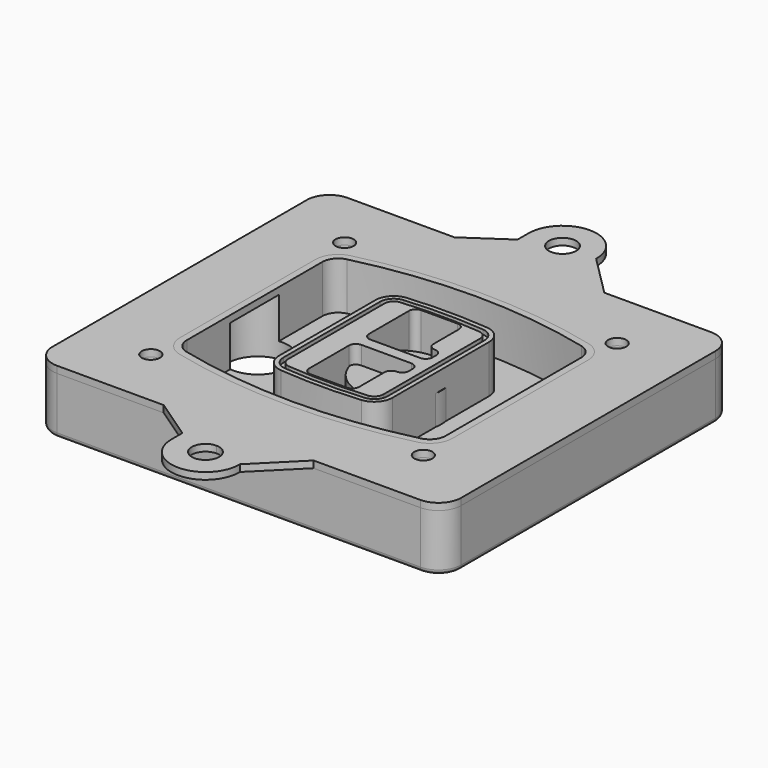
from build123d import *

# Parameters (mm, degrees)
F0_R      = 4
F1_DEPTH  = 25
F2_DEPTH  = 3
F3_DEPTH  = 18
F5_DEPTH  = 21
F6_DEPTH  = 2
F8_DEPTH  = 20
F9_DEPTH  = 16
F10_DEPTH = 25
F7_R      = 6
F7_R_2    = 4
F11_DEPTH = 6
F13_DEPTH = 9
F15_R     = 2
F16_R     = 4
F17_DEPTH = 3


# Not quite as in the source:
# - a feature of the source that left no trace in its solid (it failed there, or was rolled back) is left out
# - a feature names something its author has since deleted; it is built from what else it names


with BuildPart() as f1:
    # F0 (on Top) → F1 (new body)
    with BuildSketch(Plane.XY):
        with BuildLine():
            ThreePointArc((-90, -70), (-87.0710678119, -77.0710678119), (-80, -80))
            Line((-80, -80), (80, -80))
            ThreePointArc((80, -80), (87.0710678119, -77.0710678119), (90, -70))
            Line((90, -70), (90, 70))
            ThreePointArc((90, 70), (87.0710678119, 77.0710678119), (80, 80))
            Line((80, 80), (-80, 80))
            ThreePointArc((-80, 80), (-87.0710678119, 77.0710678119), (-90, 70))
            Line((-90, 70), (-90, -70))
        make_face()
        with Locations((-60, -53.3333333333)):
            Circle(F0_R, mode=Mode.SUBTRACT)
        with Locations((60, -53.3333333333)):
            Circle(F0_R, mode=Mode.SUBTRACT)
        with BuildLine():
            ThreePointArc((-64, 37.2990447398), (-61.0143011354, 45.9411029726), (-53.3306899286, 50.8970778549))
            ThreePointArc((-53.3306899286, 50.8970778549), (0, 57.3333333333), (53.3306899286, 50.8970778549))
            ThreePointArc((53.3306899286, 50.8970778549), (61.0143011354, 45.9411029726), (64, 37.2990447398))
            Line((64, 37.2990447398), (64, -37.2990447398))
            ThreePointArc((64, -37.2990447398), (61.0143011354, -45.9411029726), (53.3306899286, -50.8970778549))
            ThreePointArc((53.3306899286, -50.8970778549), (0, -57.3333333333), (-53.3306899286, -50.8970778549))
            ThreePointArc((-53.3306899286, -50.8970778549), (-61.0143011354, -45.9411029726), (-64, -37.2990447398))
            Line((-64, -37.2990447398), (-64, 37.2990447398))
        make_face(mode=Mode.SUBTRACT)
        with Locations((-60, 53.3333333333)):
            Circle(F0_R, mode=Mode.SUBTRACT)
        with Locations((60, 53.3333333333)):
            Circle(F0_R, mode=Mode.SUBTRACT)
        with BuildLine():
            ThreePointArc((53.3306899286, 50.8970778549), (0, 57.3333333333), (-53.3306899286, 50.8970778549))
            ThreePointArc((-53.3306899286, 50.8970778549), (-61.0143011354, 45.9411029726), (-64, 37.2990447398))
            Line((-64, 37.2990447398), (-64, -37.2990447398))
            ThreePointArc((-64, -37.2990447398), (-61.0143011354, -45.9411029726), (-53.3306899286, -50.8970778549))
            ThreePointArc((-53.3306899286, -50.8970778549), (0, -57.3333333333), (53.3306899286, -50.8970778549))
            ThreePointArc((53.3306899286, -50.8970778549), (61.0143011354, -45.9411029726), (64, -37.2990447398))
            Line((64, -37.2990447398), (64, 37.2990447398))
            ThreePointArc((64, 37.2990447398), (61.0143011354, 45.9411029726), (53.3306899286, 50.8970778549))
        make_face()
        with BuildLine():
            Line((-60, -37.2990447398), (-60, 37.2990447398))
            ThreePointArc((-60, 37.2990447398), (-57.8673579538, 43.4719434775), (-52.3790642347, 47.0119255363))
            ThreePointArc((-52.3790642347, 47.0119255363), (0, 53.3333333333), (52.3790642347, 47.0119255363))
            ThreePointArc((52.3790642347, 47.0119255363), (57.8673579538, 43.4719434775), (60, 37.2990447398))
            Line((60, 37.2990447398), (60, -37.2990447398))
            ThreePointArc((60, -37.2990447398), (57.8673579538, -43.4719434775), (52.3790642347, -47.0119255363))
            ThreePointArc((52.3790642347, -47.0119255363), (0, -53.3333333333), (-52.3790642347, -47.0119255363))
            ThreePointArc((-52.3790642347, -47.0119255363), (-57.8673579538, -43.4719434775), (-60, -37.2990447398))
        make_face(mode=Mode.SUBTRACT)
        with BuildLine():
            ThreePointArc((-52.3790642347, 47.0119255363), (-57.8673579538, 43.4719434775), (-60, 37.2990447398))
            Line((-60, 37.2990447398), (-60, -37.2990447398))
            ThreePointArc((-60, -37.2990447398), (-57.8673579538, -43.4719434775), (-52.3790642347, -47.0119255363))
            ThreePointArc((-52.3790642347, -47.0119255363), (0, -53.3333333333), (52.3790642347, -47.0119255363))
            ThreePointArc((52.3790642347, -47.0119255363), (57.8673579538, -43.4719434775), (60, -37.2990447398))
            Line((60, -37.2990447398), (60, 37.2990447398))
            ThreePointArc((60, 37.2990447398), (57.8673579538, 43.4719434775), (52.3790642347, 47.0119255363))
            ThreePointArc((52.3790642347, 47.0119255363), (0, 53.3333333333), (-52.3790642347, 47.0119255363))
        make_face()
        with BuildLine():
            ThreePointArc((51.6653449643, 44.0980612973), (55.5071505677, 41.6200738562), (57, 37.2990447398))
            Line((57, 37.2990447398), (57, -37.2990447398))
            ThreePointArc((57, -37.2990447398), (55.5071505677, -41.6200738562), (51.6653449643, -44.0980612973))
            ThreePointArc((51.6653449643, -44.0980612973), (0, -50.3333333333), (-51.6653449643, -44.0980612973))
            ThreePointArc((-51.6653449643, -44.0980612973), (-55.5071505677, -41.6200738562), (-57, -37.2990447398))
            Line((-57, -37.2990447398), (-57, 37.2990447398))
            ThreePointArc((-57, 37.2990447398), (-55.5071505677, 41.6200738562), (-51.6653449643, 44.0980612973))
            ThreePointArc((-51.6653449643, 44.0980612973), (0, 50.3333333333), (51.6653449643, 44.0980612973))
        make_face(mode=Mode.SUBTRACT)
        with BuildLine():
            Line((57, -37.2990447398), (57, 37.2990447398))
            ThreePointArc((57, 37.2990447398), (55.5071505677, 41.6200738562), (51.6653449643, 44.0980612973))
            ThreePointArc((51.6653449643, 44.0980612973), (0, 50.3333333333), (-51.6653449643, 44.0980612973))
            ThreePointArc((-51.6653449643, 44.0980612973), (-55.5071505677, 41.6200738562), (-57, 37.2990447398))
            Line((-57, 37.2990447398), (-57, -37.2990447398))
            ThreePointArc((-57, -37.2990447398), (-55.5071505677, -41.6200738562), (-51.6653449643, -44.0980612973))
            ThreePointArc((-51.6653449643, -44.0980612973), (0, -50.3333333333), (51.6653449643, -44.0980612973))
            ThreePointArc((51.6653449643, -44.0980612973), (55.5071505677, -41.6200738562), (57, -37.2990447398))
        make_face()
    extrude(amount=-F1_DEPTH)

    # F0 (on Top) → F2 (join)
    with BuildSketch(Plane.XY):
        with BuildLine():
            ThreePointArc((-52.3790642347, 47.0119255363), (-57.8673579538, 43.4719434775), (-60, 37.2990447398))
            Line((-60, 37.2990447398), (-60, -37.2990447398))
            ThreePointArc((-60, -37.2990447398), (-57.8673579538, -43.4719434775), (-52.3790642347, -47.0119255363))
            ThreePointArc((-52.3790642347, -47.0119255363), (0, -53.3333333333), (52.3790642347, -47.0119255363))
            ThreePointArc((52.3790642347, -47.0119255363), (57.8673579538, -43.4719434775), (60, -37.2990447398))
            Line((60, -37.2990447398), (60, 37.2990447398))
            ThreePointArc((60, 37.2990447398), (57.8673579538, 43.4719434775), (52.3790642347, 47.0119255363))
            ThreePointArc((52.3790642347, 47.0119255363), (0, 53.3333333333), (-52.3790642347, 47.0119255363))
        make_face()
        with BuildLine():
            ThreePointArc((51.6653449643, 44.0980612973), (55.5071505677, 41.6200738562), (57, 37.2990447398))
            Line((57, 37.2990447398), (57, -37.2990447398))
            ThreePointArc((57, -37.2990447398), (55.5071505677, -41.6200738562), (51.6653449643, -44.0980612973))
            ThreePointArc((51.6653449643, -44.0980612973), (0, -50.3333333333), (-51.6653449643, -44.0980612973))
            ThreePointArc((-51.6653449643, -44.0980612973), (-55.5071505677, -41.6200738562), (-57, -37.2990447398))
            Line((-57, -37.2990447398), (-57, 37.2990447398))
            ThreePointArc((-57, 37.2990447398), (-55.5071505677, 41.6200738562), (-51.6653449643, 44.0980612973))
            ThreePointArc((-51.6653449643, 44.0980612973), (0, 50.3333333333), (51.6653449643, 44.0980612973))
        make_face(mode=Mode.SUBTRACT)
    extrude(amount=F2_DEPTH)

    # F0 (on Top) → F3 (cut)
    with BuildSketch(Plane.XY):
        with BuildLine():
            Line((57, -37.2990447398), (57, 37.2990447398))
            ThreePointArc((57, 37.2990447398), (55.5071505677, 41.6200738562), (51.6653449643, 44.0980612973))
            ThreePointArc((51.6653449643, 44.0980612973), (0, 50.3333333333), (-51.6653449643, 44.0980612973))
            ThreePointArc((-51.6653449643, 44.0980612973), (-55.5071505677, 41.6200738562), (-57, 37.2990447398))
            Line((-57, 37.2990447398), (-57, -37.2990447398))
            ThreePointArc((-57, -37.2990447398), (-55.5071505677, -41.6200738562), (-51.6653449643, -44.0980612973))
            ThreePointArc((-51.6653449643, -44.0980612973), (0, -50.3333333333), (51.6653449643, -44.0980612973))
            ThreePointArc((51.6653449643, -44.0980612973), (55.5071505677, -41.6200738562), (57, -37.2990447398))
        make_face()
    extrude(amount=-F3_DEPTH, mode=Mode.SUBTRACT)

    # F4 (on face) → F5 (join, through all)
    with BuildSketch(Plane.XY.offset(3)):
        with BuildLine():
            ThreePointArc((-25, -26.587695628), (-22.8992979869, -31.9912392117), (-17.7004291845, -34.5569740744))
            ThreePointArc((-17.7004291845, -34.5569740744), (0, -35.3333333333), (17.7004291845, -34.5569740744))
            ThreePointArc((17.7004291845, -34.5569740744), (22.8992979869, -31.9912392117), (25, -26.587695628))
            Line((25, -26.587695628), (25, 26.587695628))
            ThreePointArc((25, 26.587695628), (22.8992979869, 31.9912392117), (17.7004291845, 34.5569740744))
            ThreePointArc((17.7004291845, 34.5569740744), (0, 35.3333333333), (-17.7004291845, 34.5569740744))
            ThreePointArc((-17.7004291845, 34.5569740744), (-22.8992979869, 31.9912392117), (-25, 26.587695628))
            Line((-25, 26.587695628), (-25, -26.587695628))
        make_face()
        with BuildLine():
            ThreePointArc((17.5253218884, 32.5646544628), (21.4244734902, 30.6403533158), (23, 26.587695628))
            Line((23, 26.587695628), (23, -26.587695628))
            ThreePointArc((23, -26.587695628), (21.4244734902, -30.6403533158), (17.5253218884, -32.5646544628))
            ThreePointArc((17.5253218884, -32.5646544628), (0, -33.3333333333), (-17.5253218884, -32.5646544628))
            ThreePointArc((-17.5253218884, -32.5646544628), (-21.4244734902, -30.6403533158), (-23, -26.587695628))
            Line((-23, -26.587695628), (-23, 26.587695628))
            ThreePointArc((-23, 26.587695628), (-21.4244734902, 30.6403533158), (-17.5253218884, 32.5646544628))
            ThreePointArc((-17.5253218884, 32.5646544628), (0, 33.3333333333), (17.5253218884, 32.5646544628))
        make_face(mode=Mode.SUBTRACT)
        with BuildLine():
            Line((23, -26.587695628), (23, 26.587695628))
            ThreePointArc((23, 26.587695628), (21.4244734902, 30.6403533158), (17.5253218884, 32.5646544628))
            ThreePointArc((17.5253218884, 32.5646544628), (0, 33.3333333333), (-17.5253218884, 32.5646544628))
            ThreePointArc((-17.5253218884, 32.5646544628), (-21.4244734902, 30.6403533158), (-23, 26.587695628))
            Line((-23, 26.587695628), (-23, -26.587695628))
            ThreePointArc((-23, -26.587695628), (-21.4244734902, -30.6403533158), (-17.5253218884, -32.5646544628))
            ThreePointArc((-17.5253218884, -32.5646544628), (0, -33.3333333333), (17.5253218884, -32.5646544628))
            ThreePointArc((17.5253218884, -32.5646544628), (21.4244734902, -30.6403533158), (23, -26.587695628))
        make_face()
        with BuildLine():
            ThreePointArc((17.3502145923, 30.5723348512), (19.9496489934, 29.2894674198), (21, 26.587695628))
            Line((21, 26.587695628), (21, -26.587695628))
            ThreePointArc((21, -26.587695628), (19.9496489934, -29.2894674198), (17.3502145923, -30.5723348512))
            ThreePointArc((17.3502145923, -30.5723348512), (0, -31.3333333333), (-17.3502145923, -30.5723348512))
            ThreePointArc((-17.3502145923, -30.5723348512), (-19.9496489934, -29.2894674198), (-21, -26.587695628))
            Line((-21, -26.587695628), (-21, 26.587695628))
            ThreePointArc((-21, 26.587695628), (-19.9496489934, 29.2894674198), (-17.3502145923, 30.5723348512))
            ThreePointArc((-17.3502145923, 30.5723348512), (0, 31.3333333333), (17.3502145923, 30.5723348512))
        make_face(mode=Mode.SUBTRACT)
        with BuildLine():
            Line((21, -26.587695628), (21, 26.587695628))
            ThreePointArc((21, 26.587695628), (19.9496489934, 29.2894674198), (17.3502145923, 30.5723348512))
            ThreePointArc((17.3502145923, 30.5723348512), (0, 31.3333333333), (-17.3502145923, 30.5723348512))
            ThreePointArc((-17.3502145923, 30.5723348512), (-19.9496489934, 29.2894674198), (-21, 26.587695628))
            Line((-21, 26.587695628), (-21, -26.587695628))
            ThreePointArc((-21, -26.587695628), (-19.9496489934, -29.2894674198), (-17.3502145923, -30.5723348512))
            ThreePointArc((-17.3502145923, -30.5723348512), (0, -31.3333333333), (17.3502145923, -30.5723348512))
            ThreePointArc((17.3502145923, -30.5723348512), (19.9496489934, -29.2894674198), (21, -26.587695628))
        make_face()
        with BuildLine():
            Line((-8, -2.5), (14, -2.5))
            ThreePointArc((14, -2.5), (16.1213203436, -3.3786796564), (17, -5.5))
            Line((17, -5.5), (17, -7.5))
            ThreePointArc((17, -7.5), (16.1213203436, -9.6213203436), (14, -10.5))
            ThreePointArc((14, -10.5), (11.8786796564, -11.3786796564), (11, -13.5))
            Line((11, -13.5), (11, -27.5))
            ThreePointArc((11, -27.5), (10.1213203436, -29.6213203436), (8, -30.5))
            Line((8, -30.5), (-8, -30.5))
            ThreePointArc((-8, -30.5), (-10.1213203436, -29.6213203436), (-11, -27.5))
            Line((-11, -27.5), (-11, -5.5))
            ThreePointArc((-11, -5.5), (-10.1213203436, -3.3786796564), (-8, -2.5))
        make_face(mode=Mode.SUBTRACT)
        with BuildLine():
            ThreePointArc((-8, 2.5), (-10.1213203436, 3.3786796564), (-11, 5.5))
            Line((-11, 5.5), (-11, 27.5))
            ThreePointArc((-11, 27.5), (-10.1213203436, 29.6213203436), (-8, 30.5))
            Line((-8, 30.5), (8, 30.5))
            ThreePointArc((8, 30.5), (10.1213203436, 29.6213203436), (11, 27.5))
            Line((11, 27.5), (11, 13.5))
            ThreePointArc((11, 13.5), (11.8786796564, 11.3786796564), (14, 10.5))
            ThreePointArc((14, 10.5), (16.1213203436, 9.6213203436), (17, 7.5))
            Line((17, 7.5), (17, 5.5))
            ThreePointArc((17, 5.5), (16.1213203436, 3.3786796564), (14, 2.5))
            Line((14, 2.5), (-8, 2.5))
        make_face(mode=Mode.SUBTRACT)
    extrude(amount=-F5_DEPTH)

    # F4 (on face) → F6 (cut)
    with BuildSketch(Plane.XY.offset(3)):
        with BuildLine():
            Line((23, -26.587695628), (23, 26.587695628))
            ThreePointArc((23, 26.587695628), (21.4244734902, 30.6403533158), (17.5253218884, 32.5646544628))
            ThreePointArc((17.5253218884, 32.5646544628), (0, 33.3333333333), (-17.5253218884, 32.5646544628))
            ThreePointArc((-17.5253218884, 32.5646544628), (-21.4244734902, 30.6403533158), (-23, 26.587695628))
            Line((-23, 26.587695628), (-23, -26.587695628))
            ThreePointArc((-23, -26.587695628), (-21.4244734902, -30.6403533158), (-17.5253218884, -32.5646544628))
            ThreePointArc((-17.5253218884, -32.5646544628), (0, -33.3333333333), (17.5253218884, -32.5646544628))
            ThreePointArc((17.5253218884, -32.5646544628), (21.4244734902, -30.6403533158), (23, -26.587695628))
        make_face()
        with BuildLine():
            ThreePointArc((17.3502145923, 30.5723348512), (19.9496489934, 29.2894674198), (21, 26.587695628))
            Line((21, 26.587695628), (21, -26.587695628))
            ThreePointArc((21, -26.587695628), (19.9496489934, -29.2894674198), (17.3502145923, -30.5723348512))
            ThreePointArc((17.3502145923, -30.5723348512), (0, -31.3333333333), (-17.3502145923, -30.5723348512))
            ThreePointArc((-17.3502145923, -30.5723348512), (-19.9496489934, -29.2894674198), (-21, -26.587695628))
            Line((-21, -26.587695628), (-21, 26.587695628))
            ThreePointArc((-21, 26.587695628), (-19.9496489934, 29.2894674198), (-17.3502145923, 30.5723348512))
            ThreePointArc((-17.3502145923, 30.5723348512), (0, 31.3333333333), (17.3502145923, 30.5723348512))
        make_face(mode=Mode.SUBTRACT)
    extrude(amount=-F6_DEPTH, mode=Mode.SUBTRACT)

    # F7 (on face) → F8 (join)
    with BuildSketch(Plane(origin=(0, 0, -25), x_dir=(1, 0, 0), z_dir=(0, 0, -1))):
        with BuildLine():
            ThreePointArc((-6.71157564, 0), (6.7567035675, 13.4682792075), (20.224982775, 0))
            Line((20.224982775, 0), (25.224982775, 0))
            ThreePointArc((25.224982775, 0), (6.7567035675, 18.4682792075), (-11.71157564, 0))
            Line((-11.71157564, 0), (-6.71157564, 0))
        make_face()
        with BuildLine():
            Line((-6.71157564, 0), (20.224982775, 0))
            ThreePointArc((20.224982775, 0), (6.7567035675, 13.4682792075), (-6.71157564, 0))
        make_face()
        with BuildLine():
            ThreePointArc((-6.71157564, 0), (6.7567035675, -13.4682792075), (20.224982775, 0))
            Line((20.224982775, 0), (-6.71157564, 0))
        make_face()
        with BuildLine():
            Line((25.224982775, 0), (20.224982775, 0))
            ThreePointArc((20.224982775, 0), (6.7567035675, -13.4682792075), (-6.71157564, 0))
            Line((-6.71157564, 0), (-11.71157564, 0))
            ThreePointArc((-11.71157564, 0), (6.7567035675, -18.4682792075), (25.224982775, 0))
        make_face()
    extrude(amount=-F8_DEPTH)

    # F7 (on face) → F9 (cut)
    with BuildSketch(Plane(origin=(0, 0, -25), x_dir=(1, 0, 0), z_dir=(0, 0, -1))):
        with BuildLine():
            Line((-6.71157564, 0), (20.224982775, 0))
            ThreePointArc((20.224982775, 0), (6.7567035675, 13.4682792075), (-6.71157564, 0))
        make_face()
        with BuildLine():
            ThreePointArc((-6.71157564, 0), (6.7567035675, -13.4682792075), (20.224982775, 0))
            Line((20.224982775, 0), (-6.71157564, 0))
        make_face()
    extrude(amount=-F9_DEPTH, mode=Mode.SUBTRACT)

    # F7 (on face) → F10 (cut)
    with BuildSketch(Plane(origin=(0, 0, -25), x_dir=(1, 0, 0), z_dir=(0, 0, -1))):
        with BuildLine():
            Line((-69.0318229325, 0), (-42.0952645175, 0))
            ThreePointArc((-42.0952645175, 0), (-55.563543725, 13.4682792075), (-69.0318229325, 0))
        make_face()
        with BuildLine():
            ThreePointArc((-69.0318229325, 0), (-55.563543725, -13.4682792075), (-42.0952645175, 0))
            Line((-42.0952645175, 0), (-69.0318229325, 0))
        make_face()
    extrude(amount=-F10_DEPTH, mode=Mode.SUBTRACT)

    # F7 (on face) → F11 (cut)
    with BuildSketch(Plane(origin=(0, 0, -25), x_dir=(1, 0, 0), z_dir=(0, 0, -1))):
        with Locations((60, -53.3333333333)):
            Circle(F7_R)
        with Locations((60, -53.3333333333)):
            Circle(F7_R_2, mode=Mode.SUBTRACT)
        with Locations((-60, -53.3333333333)):
            Circle(F7_R)
        with Locations((-60, -53.3333333333)):
            Circle(F7_R_2, mode=Mode.SUBTRACT)
        with Locations((-60, 53.3333333333)):
            Circle(F7_R)
        with Locations((-60, 53.3333333333)):
            Circle(F7_R_2, mode=Mode.SUBTRACT)
        with Locations((60, 53.3333333333)):
            Circle(F7_R)
        with Locations((60, 53.3333333333)):
            Circle(F7_R_2, mode=Mode.SUBTRACT)
    extrude(amount=-F11_DEPTH, mode=Mode.SUBTRACT)

    # F12 (on face) → F13 (cut, through all)
    with BuildSketch(Plane(origin=(0, 0, -9), x_dir=(1, 0, 0), z_dir=(0, 0, -1))):
        with BuildLine():
            ThreePointArc((20.224982775, 0), (20.1663399806, 1.2554664788), (19.9909222755, 2.5))
            Line((19.9909222755, 2.5), (14, 2.5))
            ThreePointArc((14, 2.5), (16.1213203436, 3.3786796564), (17, 5.5))
            Line((17, 5.5), (17, 7.5))
            ThreePointArc((17, 7.5), (16.1213203436, 9.6213203436), (14, 10.5))
            ThreePointArc((14, 10.5), (12.1627255951, 11.1284134507), (11.0951631559, 12.750384826))
            ThreePointArc((11.0951631559, 12.750384826), (11.0476113807, 12.7664660322), (11, 12.7823698976))
            Line((11, 12.7823698976), (11, -12.7823698976))
            ThreePointArc((11, -12.7823698976), (11.0476113807, -12.7664660322), (11.0951631559, -12.750384826))
            ThreePointArc((11.0951631559, -12.750384826), (12.1627255951, -11.1284134507), (14, -10.5))
            ThreePointArc((14, -10.5), (16.1213203436, -9.6213203436), (17, -7.5))
            Line((17, -7.5), (17, -5.5))
            ThreePointArc((17, -5.5), (16.1213203436, -3.3786796564), (14, -2.5))
            Line((14, -2.5), (19.9909222755, -2.5))
            ThreePointArc((19.9909222755, -2.5), (20.1663399806, -1.2554664788), (20.224982775, 0))
        make_face()
    extrude(amount=F13_DEPTH, mode=Mode.SUBTRACT)

    # F15
    f15_edges = [f1.edges().sort_by_distance(p)[0] for p in [
        (0, -80, -25),
        (-87.071068, -77.071068, -25),
        (-90, 0, -25),
        (-87.071068, 77.071068, -25),
        (87.071068, -77.071068, -25),
        (0, 80, -25),
        (90, 0, -25),
        (87.071068, 77.071068, -25),
    ]]
    fillet(f15_edges, radius=F15_R)


with BuildPart() as f17:
    # F16 (on face) → F17 (new body, through all)
    with BuildSketch(Plane.XY):
        with BuildLine():
            Line((-33, 80), (-80, 80))
            ThreePointArc((-80, 80), (-87.0710678119, 77.0710678119), (-90, 70))
            Line((-90, 70), (-90, -70))
            ThreePointArc((-90, -70), (-87.0710678119, -77.0710678119), (-80, -80))
            Line((-80, -80), (-33, -80))
            Line((-33, -80), (0, -80))
            Line((0, -80), (33, -80))
            Line((33, -80), (80, -80))
            ThreePointArc((80, -80), (87.0710678119, -77.0710678119), (90, -70))
            Line((90, -70), (90, 70))
            ThreePointArc((90, 70), (87.0710678119, 77.0710678119), (80, 80))
            Line((80, 80), (33, 80))
            Line((33, 80), (0, 80))
            Line((0, 80), (-33, 80))
        make_face()
        with Locations((-60, -53.3333333333)):
            Circle(F16_R, mode=Mode.SUBTRACT)
        with BuildLine():
            ThreePointArc((52.3790642347, -47.0119255363), (0, -53.3333333333), (-52.3790642347, -47.0119255363))
            ThreePointArc((-52.3790642347, -47.0119255363), (-57.8673579538, -43.4719434775), (-60, -37.2990447398))
            Line((-60, -37.2990447398), (-60, 37.2990447398))
            ThreePointArc((-60, 37.2990447398), (-57.8673579538, 43.4719434775), (-52.3790642347, 47.0119255363))
            ThreePointArc((-52.3790642347, 47.0119255363), (0, 53.3333333333), (52.3790642347, 47.0119255363))
            ThreePointArc((52.3790642347, 47.0119255363), (57.8673579538, 43.4719434775), (60, 37.2990447398))
            Line((60, 37.2990447398), (60, -37.2990447398))
            ThreePointArc((60, -37.2990447398), (57.8673579538, -43.4719434775), (52.3790642347, -47.0119255363))
        make_face(mode=Mode.SUBTRACT)
        with Locations((60, -53.3333333333)):
            Circle(F16_R, mode=Mode.SUBTRACT)
        with Locations((-60, 53.3333333333)):
            Circle(F16_R, mode=Mode.SUBTRACT)
        with Locations((60, 53.3333333333)):
            Circle(F16_R, mode=Mode.SUBTRACT)
        with BuildLine():
            Line((-15, 92.25), (-33, 80))
            Line((-33, 80), (0, 80))
            Line((0, 80), (33, 80))
            Line((33, 80), (15, 98))
            Line((15, 98), (15, 98.25))
            ThreePointArc((15, 98.25), (0, 113.25), (-15, 98.25))
            Line((-15, 98.25), (-15, 92.25))
        make_face()
        with BuildLine():
            ThreePointArc((6, 98.25), (4.2426406871, 94.0073593129), (0, 92.25))
            ThreePointArc((0, 92.25), (-4.2426406871, 102.4926406871), (6, 98.25))
        make_face(mode=Mode.SUBTRACT)
        with BuildLine():
            Line((0, -80), (-33, -80))
            Line((-33, -80), (-15, -92.25))
            Line((-15, -92.25), (-15, -98.25))
            ThreePointArc((-15, -98.25), (0, -113.25), (15, -98.25))
            Line((15, -98.25), (15, -98))
            Line((15, -98), (33, -80))
            Line((33, -80), (0, -80))
        make_face()
        with BuildLine():
            ThreePointArc((6, -98.25), (-4.2426406871, -102.4926406871), (0, -92.25))
            ThreePointArc((0, -92.25), (4.2426406871, -94.0073593129), (6, -98.25))
        make_face(mode=Mode.SUBTRACT)
    extrude(amount=F17_DEPTH)


solid = Compound([f1.part, f17.part])
